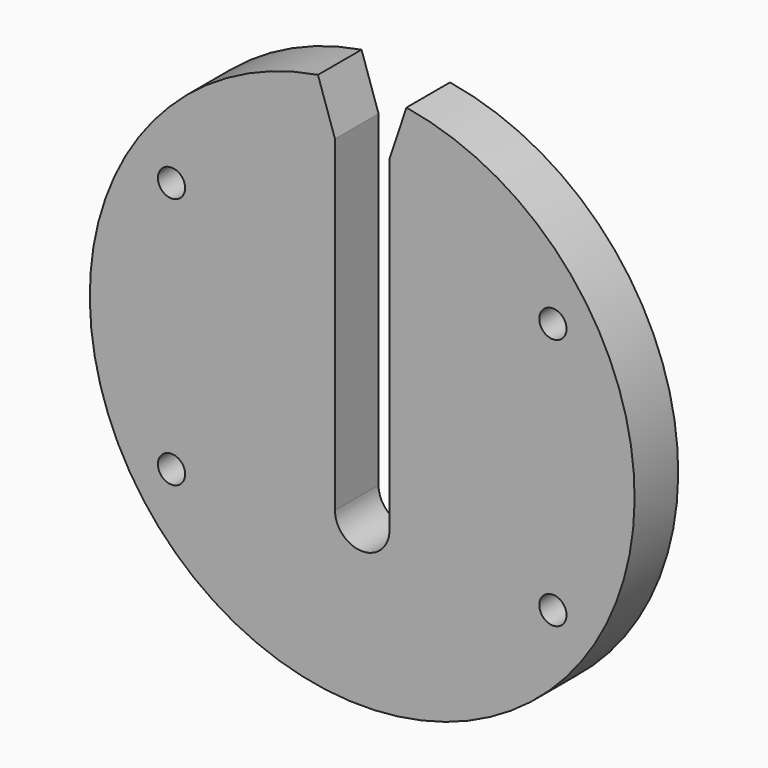
from build123d import *

# Parameters (mm, degrees)
F0_R           = 63.5
F1_DEPTH       = 12.7
F3_DEPTH       = 25.4
F4_D           = 6.35
F4_CBORE_D     = 10.3124
F4_CBORE_DEPTH = 6.35


# Not quite as in the source:
# - a feature names something its author has since deleted; it is built from what else it names


with BuildPart() as f1:
    # F0 (on Front) → F1 (new body)
    with BuildSketch(Plane.XZ):
        Circle(F0_R)
    extrude(amount=F1_DEPTH)

    # F2 (on face) → F3 (cut)
    with BuildSketch(Plane.XZ.offset(12.7)):
        with BuildLine():
            Line((-10.3124, 62.6570379625), (-6.35, 50.8))
            Line((-6.35, 50.8), (-6.35, -25.4))
            ThreePointArc((-6.35, -25.4), (0, -31.75), (6.35, -25.4))
            Line((6.35, -25.4), (6.35, 50.8))
            Line((6.35, 50.8), (10.3124, 62.6570379625))
            ThreePointArc((10.3124, 62.6570379625), (0, 63.5), (-10.3124, 62.6570379625))
        make_face()
    extrude(amount=-F3_DEPTH, mode=Mode.SUBTRACT)

    # F4 (through all)
    with Locations(Plane(origin=(0, 0, 0), x_dir=(1, 0, 0), z_dir=(0, 1, 0))):
        with Locations((44.45, -29.36875), (-44.45, -29.36875), (44.45, 29.36875), (-44.45, 29.36875)):
            CounterBoreHole(F4_D / 2, F4_CBORE_D / 2, F4_CBORE_DEPTH)


solid = f1.part
